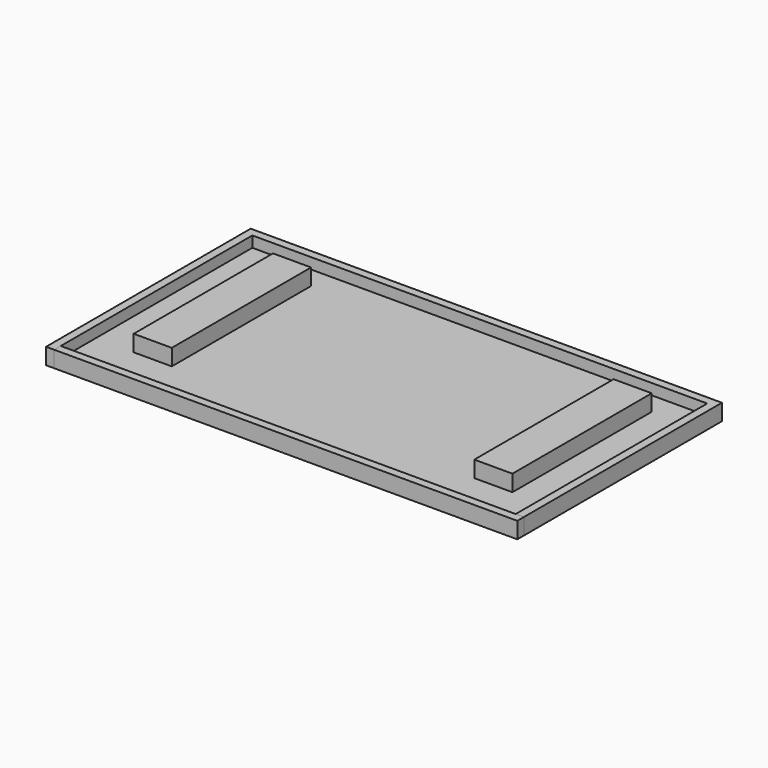
from build123d import *

# Parameters (mm, degrees)
F0_W     = 1061.72
F0_H     = 558.8
F1_DEPTH = 6.35
F2_W     = 19.05
F2_H     = 38.1
F3_DEPTH = 1080.77
F4_W     = 19.05
F4_H     = 38.1
F5_DEPTH = 596.9
F6_W     = 88.9
F6_H     = 406.4
F7_DEPTH = 38.1


with BuildPart() as f1:
    # F0 (on Top) → F1 (new body)
    with BuildSketch(Plane.XY):
        with Locations((476.4319329417, 228.4453787148)):
            Rectangle(F0_W, F0_H)
    extrude(amount=F1_DEPTH)

    # F6 (on face) → F7 (join)
    with BuildSketch(Plane.XY.offset(6.35)):
        with Locations((78.9219329417, 253.8453787148)):
            Rectangle(F6_W, F6_H)
        with Locations((873.9419329417, 253.8453787148)):
            Rectangle(F6_W, F6_H)
    extrude(amount=F7_DEPTH)


with BuildPart() as f3:
    # F2 (on face) → F3 (new body)
    with BuildSketch(Plane(origin=(-54.4280670583, 0, 0), x_dir=(0, -1, 0), z_dir=(-1, 0, 0))):
        with Locations((-517.3703787148, 12.7)):
            Rectangle(F2_W, F2_H)
    extrude(amount=-F3_DEPTH)

    # F4 (on face) → F5 (join)
    with BuildSketch(Plane(origin=(0, 526.8953787148, 0), x_dir=(-1, 0, 0), z_dir=(0, 1, 0))):
        with Locations((-1016.8169329417, 12.7)):
            Rectangle(F4_W, F4_H)
        with Locations((63.9530670583, 12.7)):
            Rectangle(F4_W, F4_H)
    extrude(amount=-F5_DEPTH)


with BuildPart() as f3b:
    # F2 (on face) → F3, piece 2 (new body)
    with BuildSketch(Plane(origin=(-54.4280670583, 0, 0), x_dir=(0, -1, 0), z_dir=(-1, 0, 0))):
        with Locations((60.4796212852, 12.7)):
            Rectangle(F2_W, F2_H)
    extrude(amount=-F3_DEPTH)


solid = Compound([f1.part, f3.part, f3b.part])
